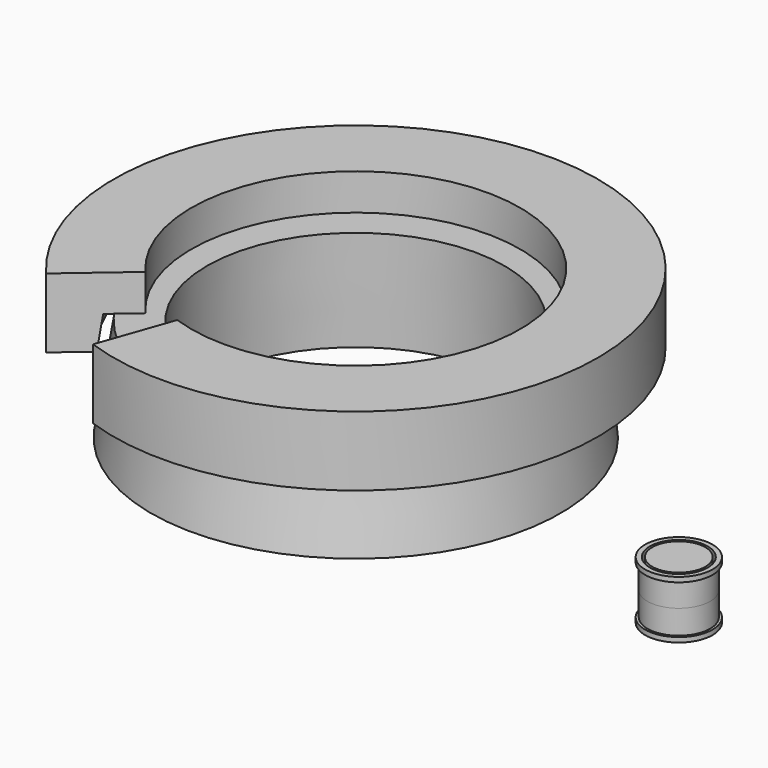
from build123d import *

# Parameters (mm, degrees)
F0_R     = 6.5
F0_R_2   = 6
F1_DEPTH = 6
F0_R_3   = 7
F2_DEPTH = 1
F0_R_4   = 5.5
F4_DEPTH = 12
F9_DEPTH = 25


with BuildPart() as f1:
    # F0 (on Top) → F1 (new body)
    with BuildSketch(Plane.XY):
        Circle(F0_R)
        Circle(F0_R_2, mode=Mode.SUBTRACT)
    extrude(amount=-F1_DEPTH)

    # F0 (on Top) → F2 (join)
    with BuildSketch(Plane.XY):
        Circle(F0_R_3)
        Circle(F0_R, mode=Mode.SUBTRACT)
    extrude(amount=-F2_DEPTH)

    # F3: F1 across face


with BuildPart() as f1_1:
    add(f1.part)
    add(f1.part.mirror(Plane(origin=(0, 0, -6), x_dir=(1, 0, 0), z_dir=(0, 0, -1))))


with BuildPart() as f4:
    # F0 (on Top) → F4 (new body)
    with BuildSketch(Plane.XY):
        Circle(F0_R_4)
    extrude(amount=-F4_DEPTH)


with BuildPart() as f6:
    # F5 (on Front) → F6 (revolve)
    with BuildSketch(Plane.XZ):
        Polygon((-109.5425453782, 0), (-98.7844988704, 0), (-97.9169787446, 21.3577989489), (-106.291412111, 21.3577989489), align=None)
    revolve(axis=Axis((-67.0425453782, 0, 15), (0, 0, 1)))


with BuildPart() as f7:
    # F5 (on Front) → F7 (revolve)
    with BuildSketch(Plane.XZ):
        Polygon((-117.2685921192, 16.4775380677), (-109.0573355747, 16.4775380677), (-108.2686355544, 21.658776448), (-108.0100064425, 23.3577989489), (-106.291412111, 23.3577989489), (-101.1670082808, 23.3577989489), (-101.1670082808, 30.9135392308), (-117.2685921192, 30.9135392308), align=None)
    revolve(axis=Axis((-67.0425453782, 0, 15), (0, 0, 1)))

    # F8 (on face) → F9 (cut)
    with BuildSketch(Plane.XY.offset(30.9135392308)):
        with BuildLine():
            ThreePointArc((-78.3358060439, -32.2015718859), (-86.2853776046, -28.1814189901), (-92.9235819492, -22.2407489621))
            Line((-92.9235819492, -22.2407489621), (-105.1355156979, -32.7350176944))
            ThreePointArc((-105.1355156979, -32.7350176944), (-95.365083189, -41.4787852183), (-83.6645165335, -47.3958420765))
            Line((-83.6645165335, -47.3958420765), (-78.3358060439, -32.2015718859))
        make_face()
    extrude(amount=-F9_DEPTH, mode=Mode.SUBTRACT)


solid = Compound([f1_1.part, f4.part, f6.part, f7.part])
